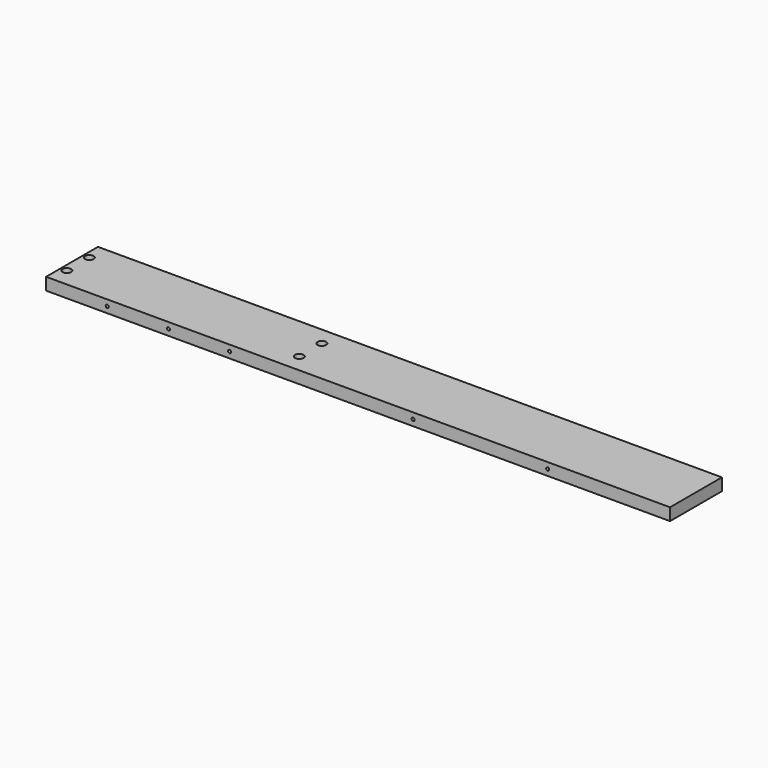
from build123d import *

# Parameters (mm, degrees)
F0_W           = 10
F0_H           = 53
F0_W_2         = 180
F0_W_3         = 310
F1_DEPTH       = 10
F3_D           = 3.5
F3_CBORE_D     = 7
F3_CBORE_DEPTH = 5
F4_R           = 1.25
F5_DEPTH       = 53


# Not quite as in the source:
# - a feature names something its author has since deleted; it is built from what else it names


with BuildPart() as f1:
    # F0 (on Top) → F1 (new body)
    with BuildSketch(Plane.XY):
        with Locations((-224.1861552, -33.3002303571)):
            Rectangle(F0_W, F0_H)
        with Locations((-129.1861552, -33.3002303571)):
            Rectangle(F0_W_2, F0_H)
        with Locations((-34.1861552, -33.3002303571)):
            Rectangle(F0_W, F0_H)
        with Locations((125.8138448, -33.3002303571)):
            Rectangle(F0_W_3, F0_H)
    extrude(amount=F1_DEPTH)

    # F3 (through all)
    with Locations(Plane.XY.offset(10)):
        with Locations((-224.1861552, -21.8002303571), (-224.1861552, -44.8002303571), (-34.1861620545, -21.8002303571), (-34.1861620545, -44.8002303571)):
            CounterBoreHole(F3_D / 2, F3_CBORE_D / 2, F3_CBORE_DEPTH)

    # F4 (on face) → F5 (cut, through all)
    with BuildSketch(Plane(origin=(0, -6.8002303571, 0), x_dir=(-1, 0, 0), z_dir=(0, 1, 0))):
        with Locations((-180.8138448, 5)):
            Circle(F4_R)
        with Locations((-70.8138448, 5)):
            Circle(F4_R)
        with Locations((79.1861552, 5)):
            Circle(F4_R)
        with Locations((129.1861552, 5)):
            Circle(F4_R)
        with Locations((179.1861552, 5)):
            Circle(F4_R)
    extrude(amount=-F5_DEPTH, mode=Mode.SUBTRACT)


solid = f1.part
